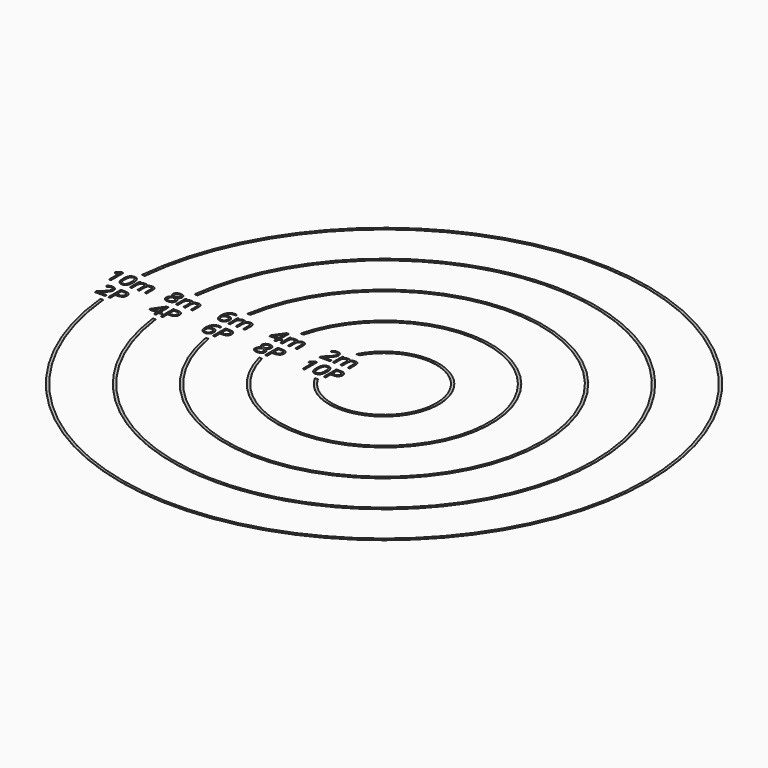
from build123d import *

# Parameters (mm, degrees)
F0_R         = 10100
F0_R_2       = 10000
F1_DEPTH     = 10
F0_R_3       = 8100
F0_R_4       = 8000
F0_R_5       = 6100
F0_R_6       = 6000
F0_R_7       = 4100
F0_R_8       = 4000
F0_R_9       = 2100
F0_R_10      = 2000
F2_W         = 12000
F2_H         = 2000
F3_DEPTH     = 10.001
F4_TEXT_SIZE = 833.3333333333
F5_DEPTH     = 10


# Not quite as in the source:
# - Text() gives the source's letters only with a copy of the font that has no kerning and outlines rounded to 1/6400 em; it was checked with that copy


with BuildPart() as f1:
    # F0 (on Top) → F1 (new body)
    with BuildSketch(Plane.XY):
        Circle(F0_R)
        Circle(F0_R_2, mode=Mode.SUBTRACT)
    extrude(amount=F1_DEPTH)


with BuildPart() as f1b:
    # F0 (on Top) → F1, piece 2 (new body)
    with BuildSketch(Plane.XY):
        Circle(F0_R_3)
        Circle(F0_R_4, mode=Mode.SUBTRACT)
    extrude(amount=F1_DEPTH)


with BuildPart() as f1c:
    # F0 (on Top) → F1, piece 3 (new body)
    with BuildSketch(Plane.XY):
        Circle(F0_R_5)
        Circle(F0_R_6, mode=Mode.SUBTRACT)
    extrude(amount=F1_DEPTH)


with BuildPart() as f1d:
    # F0 (on Top) → F1, piece 4 (new body)
    with BuildSketch(Plane.XY):
        Circle(F0_R_7)
        Circle(F0_R_8, mode=Mode.SUBTRACT)
    extrude(amount=F1_DEPTH)


with BuildPart() as f1e:
    # F0 (on Top) → F1, piece 5 (new body)
    with BuildSketch(Plane.XY):
        Circle(F0_R_9)
        Circle(F0_R_10, mode=Mode.SUBTRACT)
    extrude(amount=F1_DEPTH)


with BuildPart() as f3_tool:
    # F2 (on Top) → F3 (new body, through all)
    with BuildSketch(Plane.XY):
        with Locations((-6000, 0)):
            Rectangle(F2_W, F2_H)
    extrude(amount=F3_DEPTH)


with BuildPart() as f1_1:
    add(f1.part)

    # F3: cut by f3_tool
    add(f3_tool.part, mode=Mode.SUBTRACT)


with BuildPart() as f1b_1:
    add(f1b.part)

    # F3: cut by f3_tool
    add(f3_tool.part, mode=Mode.SUBTRACT)


with BuildPart() as f1c_1:
    add(f1c.part)

    # F3: cut by f3_tool
    add(f3_tool.part, mode=Mode.SUBTRACT)


with BuildPart() as f1d_1:
    add(f1d.part)

    # F3: cut by f3_tool
    add(f3_tool.part, mode=Mode.SUBTRACT)


with BuildPart() as f1e_1:
    add(f1e.part)

    # F3: cut by f3_tool
    add(f3_tool.part, mode=Mode.SUBTRACT)


with BuildPart() as f5:
    # F4 (on Top) → F5 (new body, through all)
    with BuildSketch(Plane.XY):
        with Locations((-2619.0104166667, 150)):
            Text('2m', F4_TEXT_SIZE, font='Open Sans', text_align=(TextAlign.LEFT, TextAlign.BOTTOM))
        with Locations((-4619.0104166667, 150)):
            Text('4m', F4_TEXT_SIZE, font='Open Sans', text_align=(TextAlign.LEFT, TextAlign.BOTTOM))
        with Locations((-6619.0104166667, 150)):
            Text('6m', F4_TEXT_SIZE, font='Open Sans', text_align=(TextAlign.LEFT, TextAlign.BOTTOM))
        with Locations((-8619.0104166667, 150)):
            Text('8m', F4_TEXT_SIZE, font='Open Sans', text_align=(TextAlign.LEFT, TextAlign.BOTTOM))
        with Locations((-10857.2265625, 150)):
            Text('10m', F4_TEXT_SIZE, font='Open Sans', text_align=(TextAlign.LEFT, TextAlign.BOTTOM))
        with Locations((-2732.9427083333, -750)):
            Text('10P', F4_TEXT_SIZE, font='Open Sans', text_align=(TextAlign.LEFT, TextAlign.BOTTOM))
        with Locations((-4494.7265625, -750)):
            Text('8P', F4_TEXT_SIZE, font='Open Sans', text_align=(TextAlign.LEFT, TextAlign.BOTTOM))
        with Locations((-6494.7265625, -750)):
            Text('6P', F4_TEXT_SIZE, font='Open Sans', text_align=(TextAlign.LEFT, TextAlign.BOTTOM))
        with Locations((-8494.7265625, -750)):
            Text('4P', F4_TEXT_SIZE, font='Open Sans', text_align=(TextAlign.LEFT, TextAlign.BOTTOM))
        with Locations((-10494.7265625, -750)):
            Text('2P', F4_TEXT_SIZE, font='Open Sans', text_align=(TextAlign.LEFT, TextAlign.BOTTOM))
    extrude(amount=F5_DEPTH)


solid = Compound([f1_1.part, f1b_1.part, f1c_1.part, f1d_1.part, f1e_1.part, f5.part])
